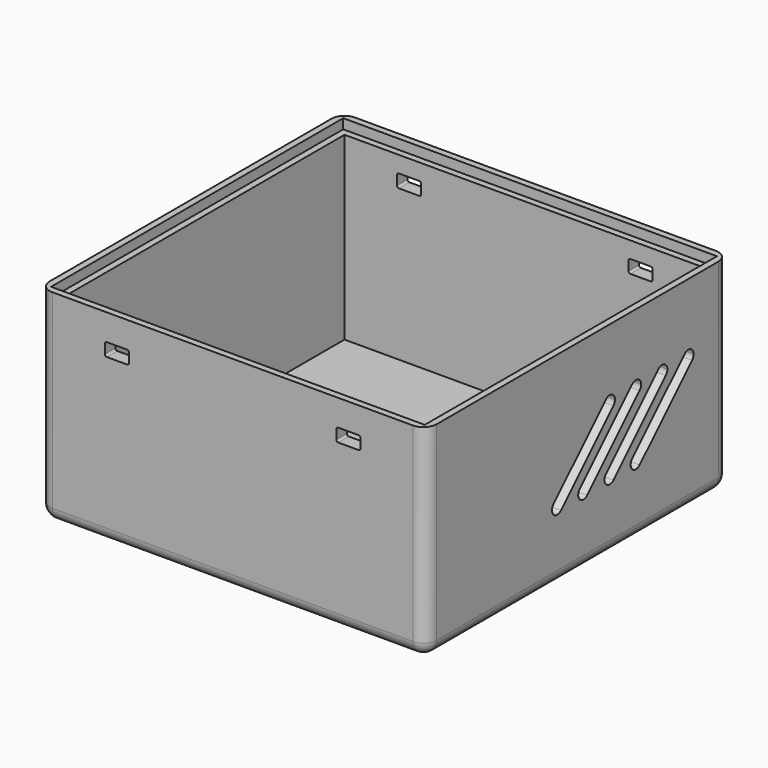
from build123d import *

# Parameters (mm, degrees)
F0_W      = 55
F0_H      = 53.7
F0_R      = 2
F1_DEPTH  = 2
F2_DEPTH  = 4
F3_W      = 55
F3_H      = 27.5
F3_W_2    = 3.7
F3_H_2    = 2
F4_DEPTH  = 2
F5_START  = 1
F3_H_3    = 1.5
F5_DEPTH  = 1
F6_W      = 53.7
F6_H      = 27.5
F7_DEPTH  = 2
F8_START  = 1
F8_DEPTH  = 1
F10_DEPTH = 1.5
F11_W     = 55
F11_H     = 27.5
F11_W_2   = 3.7
F11_H_2   = 2
F12_DEPTH = 2
F13_START = 1
F13_DEPTH = 1
F15_DEPTH = 1.5
F16_W     = 1
F16_H     = 1.5
F16_W_2   = 53.7
F16_H_2   = 27.5
F17_DEPTH = 2
F18_START = 1
F18_DEPTH = 1
F20_DEPTH = 1.5
F21_W     = 1
F21_H     = 1
F22_DEPTH = 1.5
F23_R     = 0.3
F24_R     = 2
F25_R     = 0.5


with BuildPart() as f1:
    # F0 (on Top) → F1 (new body)
    with BuildSketch(Plane.XY):
        with Locations((27.5, 26.85)):
            Rectangle(F0_W, F0_H)
        with Locations((12, 11)):
            Circle(F0_R, mode=Mode.SUBTRACT)
        with Locations((43, 11)):
            Circle(F0_R, mode=Mode.SUBTRACT)
        with Locations((27.5, 46.7)):
            Circle(F0_R, mode=Mode.SUBTRACT)
    extrude(amount=F1_DEPTH)

    # F0 (on Top) → F2 (join)
    with BuildSketch(Plane.XY):
        with Locations((12, 11)):
            Circle(F0_R)
        with Locations((27.5, 46.7)):
            Circle(F0_R)
        with Locations((43, 11)):
            Circle(F0_R)
    extrude(amount=F2_DEPTH)

    # F3 (on face) → F4 (join)
    with BuildSketch(Plane.XZ):
        with Locations((27.5, 15.75)):
            Rectangle(F3_W, F3_H)
        with Locations((9.85, 26)):
            Rectangle(F3_W_2, F3_H_2, mode=Mode.SUBTRACT)
        with Locations((45.15, 26)):
            Rectangle(F3_W_2, F3_H_2, mode=Mode.SUBTRACT)
        with Locations((27.5, 1)):
            Rectangle(F3_W, F3_H_2)
    extrude(amount=F4_DEPTH)

    # F3 (on face) → F5 (join)
    with BuildSketch(Plane.XZ.offset(F5_START)):
        with Locations((27.5, 30.25)):
            Rectangle(F3_W, F3_H_3)
    extrude(amount=F5_DEPTH)

    # F6 (on face) → F7 (join)
    with BuildSketch(Plane.YZ.offset(55)):
        Polygon((-2, 29.5), (-2, 0), (53.7, 0), (53.7, 2), (0, 2), (0, 29.5), (-1, 29.5), align=None)
        with Locations((26.85, 15.75)):
            Rectangle(F6_W, F6_H)
        with BuildLine():
            ThreePointArc((23.7071067812, 9.7928932188), (22.2928932188, 9.7928932188), (22.2928932188, 11.2071067812))
            Line((22.2928932188, 11.2071067812), (32.2928932188, 21.2071067812))
            ThreePointArc((32.2928932188, 21.2071067812), (33.3826834324, 21.4238795325), (34, 20.5))
            ThreePointArc((34, 20.5), (33.9238795325, 20.1173165676), (33.7071067812, 19.7928932188))
            Line((33.7071067812, 19.7928932188), (23.7071067812, 9.7928932188))
        make_face(mode=Mode.SUBTRACT)
        with BuildLine():
            ThreePointArc((28.7071067812, 9.7928932188), (27.2928932188, 9.7928932188), (27.2928932188, 11.2071067812))
            Line((27.2928932188, 11.2071067812), (37.2928932188, 21.2071067812))
            ThreePointArc((37.2928932188, 21.2071067812), (38.3826834324, 21.4238795325), (39, 20.5))
            ThreePointArc((39, 20.5), (38.9238795325, 20.1173165676), (38.7071067812, 19.7928932188))
            Line((38.7071067812, 19.7928932188), (28.7071067812, 9.7928932188))
        make_face(mode=Mode.SUBTRACT)
        with BuildLine():
            ThreePointArc((33.7071067812, 9.7928932188), (32.2928932188, 9.7928932188), (32.2928932188, 11.2071067812))
            Line((32.2928932188, 11.2071067812), (42.2928932188, 21.2071067812))
            ThreePointArc((42.2928932188, 21.2071067812), (43.3826834324, 21.4238795325), (44, 20.5))
            ThreePointArc((44, 20.5), (43.9238795325, 20.1173165676), (43.7071067812, 19.7928932188))
            Line((43.7071067812, 19.7928932188), (33.7071067812, 9.7928932188))
        make_face(mode=Mode.SUBTRACT)
        with BuildLine():
            ThreePointArc((38.7071067812, 9.7928932188), (37.2928932188, 9.7928932188), (37.2928932188, 11.2071067812))
            Line((37.2928932188, 11.2071067812), (47.2928932188, 21.2071067812))
            ThreePointArc((47.2928932188, 21.2071067812), (48.3826834324, 21.4238795325), (49, 20.5))
            ThreePointArc((49, 20.5), (48.9238795325, 20.1173165676), (48.7071067812, 19.7928932188))
            Line((48.7071067812, 19.7928932188), (38.7071067812, 9.7928932188))
        make_face(mode=Mode.SUBTRACT)
    extrude(amount=F7_DEPTH)

    # F6 (on face) → F8 (join)
    with BuildSketch(Plane.YZ.offset(55).offset(F8_START)):
        Polygon((-1, 31), (-1, 29.5), (0, 29.5), (53.7, 29.5), (53.7, 31), align=None)
    extrude(amount=F8_DEPTH)

    # F9 (on face) → F10 (join)
    with BuildSketch(Plane.XY.offset(29.5)):
        Polygon((56, -1), (55, -1), (55, -2), (57, -2), (57, -1), align=None)
    extrude(amount=F10_DEPTH)

    # F11 (on face) → F12 (join)
    with BuildSketch(Plane(origin=(0, 53.7, 0), x_dir=(-1, 0, 0), z_dir=(0, 1, 0))):
        with Locations((-27.5, 15.75)):
            Rectangle(F11_W, F11_H)
        with Locations((-45.15, 26)):
            Rectangle(F11_W_2, F11_H_2, mode=Mode.SUBTRACT)
        with Locations((-9.85, 26)):
            Rectangle(F11_W_2, F11_H_2, mode=Mode.SUBTRACT)
        Polygon((-57, 29.5), (-57, 0), (0, 0), (0, 2), (-55, 2), (-55, 29.5), (-56, 29.5), align=None)
    extrude(amount=F12_DEPTH)

    # F11 (on face) → F13 (join)
    with BuildSketch(Plane(origin=(0, 53.7, 0), x_dir=(-1, 0, 0), z_dir=(0, 1, 0)).offset(F13_START)):
        Polygon((-56, 31), (-56, 29.5), (-55, 29.5), (0, 29.5), (0, 31), align=None)
    extrude(amount=F13_DEPTH)

    # F14 (on face) → F15 (join)
    with BuildSketch(Plane.XY.offset(29.5)):
        Polygon((56, 54.7), (56, 53.7), (57, 53.7), (57, 55.7), (56, 55.7), align=None)
    extrude(amount=F15_DEPTH)

    # F16 (on face) → F17 (join)
    with BuildSketch(Plane(origin=(0, 0, 0), x_dir=(0, -1, 0), z_dir=(-1, 0, 0))):
        Polygon((-55.7, 29.5), (-55.7, 0), (2, 0), (2, 29.5), (1, 29.5), (0, 29.5), (0, 2), (-53.7, 2), (-53.7, 29.5), (-54.7, 29.5), align=None)
        with Locations((1.5, 30.25)):
            Rectangle(F16_W, F16_H)
        with Locations((-26.85, 15.75)):
            Rectangle(F16_W_2, F16_H_2)
    extrude(amount=F17_DEPTH)

    # F16 (on face) → F18 (join)
    with BuildSketch(Plane(origin=(0, 0, 0), x_dir=(0, -1, 0), z_dir=(-1, 0, 0)).offset(F18_START)):
        Polygon((-54.7, 31), (-54.7, 29.5), (-53.7, 29.5), (0, 29.5), (1, 29.5), (1, 31), align=None)
    extrude(amount=F18_DEPTH)

    # F19 (on face) → F20 (join)
    with BuildSketch(Plane.XY.offset(29.5)):
        Polygon((0, 54.7), (0, 55.7), (-2, 55.7), (-2, 54.7), (-1, 54.7), align=None)
    extrude(amount=F20_DEPTH)

    # F21 (on face) → F22 (join)
    with BuildSketch(Plane.XY.offset(29.5)):
        with Locations((-0.5, -1.5)):
            Rectangle(F21_W, F21_H)
    extrude(amount=F22_DEPTH)

    # F23
    f23_edges = [f1.edges().sort_by_distance(p)[0] for p in [
        (8, -1, 27),
        (11.7, -1, 27),
        (8, -1, 25),
        (11.7, -1, 25),
        (43.3, -1, 25),
        (47, -1, 25),
        (43.3, -1, 27),
        (47, -1, 27),
        (47, 54.7, 27),
        (43.3, 54.7, 25),
        (43.3, 54.7, 27),
        (47, 54.7, 25),
        (11.7, 54.7, 25),
        (8, 54.7, 25),
        (11.7, 54.7, 27),
        (8, 54.7, 27),
    ]]
    fillet(f23_edges, radius=F23_R)

    # F24
    f24_edges = [f1.edges().sort_by_distance(p)[0] for p in [
        (57, 26.85, 0),
        (27.5, 55.7, 0),
        (27.5, -2, 0),
        (-2, 26.85, 0),
        (57, -2, 15.5),
        (57, 55.7, 15.5),
        (-2, 55.7, 15.5),
        (-2, -2, 15.5),
    ]]
    fillet(f24_edges, radius=F24_R)

    # F25
    f25_edges = [f1.edges().sort_by_distance(p)[0] for p in [
        (10, 11, 4),
        (25.5, 46.7, 4),
        (41, 11, 4),
    ]]
    fillet(f25_edges, radius=F25_R)


solid = f1.part
